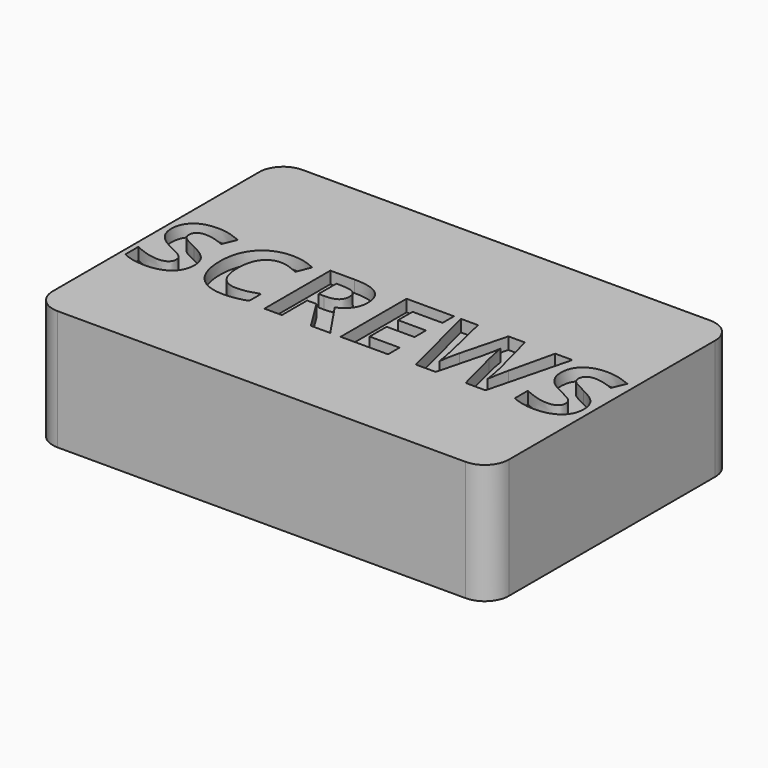
from build123d import *

# Parameters (mm, degrees)
F0_W         = 38
F0_H         = 25.5
F1_DEPTH     = 10
F2_W         = 36.3
F2_H         = 23.8
F3_DEPTH     = 5
F4_TEXT_SIZE = 9.617590066
F5_DEPTH     = 1
F6_R         = 2
F7_R         = 2


# Not quite as in the source:
# - Text() gives the source's letters only with a copy of the font that has no kerning and outlines rounded to 1/6400 em; it was checked with that copy


with BuildPart() as f1:
    # F0 (on Top) → F1 (new body)
    with BuildSketch(Plane.XY):
        Rectangle(F0_W, F0_H)
    extrude(amount=-F1_DEPTH)

    # F2 (on face) → F3 (cut)
    with BuildSketch(Plane(origin=(0, 0, -10), x_dir=(1, 0, 0), z_dir=(0, 0, -1))):
        Rectangle(F2_W, F2_H)
    extrude(amount=-F3_DEPTH, mode=Mode.SUBTRACT)

    # F4 (on face) → F5 (cut)
    with BuildSketch(Plane.XY):
        with Locations((-19, -4.0680003241)):
            Text('SCREWS', F4_TEXT_SIZE, font='Open Sans', font_style=FontStyle.BOLD, text_align=(TextAlign.LEFT, TextAlign.BOTTOM))
    extrude(amount=-F5_DEPTH, mode=Mode.SUBTRACT)

    # F6
    f6_edges = [f1.edges().sort_by_distance(p)[0] for p in [
        (-19, -12.75, -5),
        (19, -12.75, -5),
        (19, 12.75, -5),
        (-19, 12.75, -5),
    ]]
    fillet(f6_edges, radius=F6_R)

    # F7
    f7_edges = [f1.edges().sort_by_distance(p)[0] for p in [
        (18.15, -11.9, -7.5),
        (-18.15, -11.9, -7.5),
        (-18.15, 11.9, -7.5),
        (18.15, 11.9, -7.5),
    ]]
    fillet(f7_edges, radius=F7_R)


solid = f1.part
